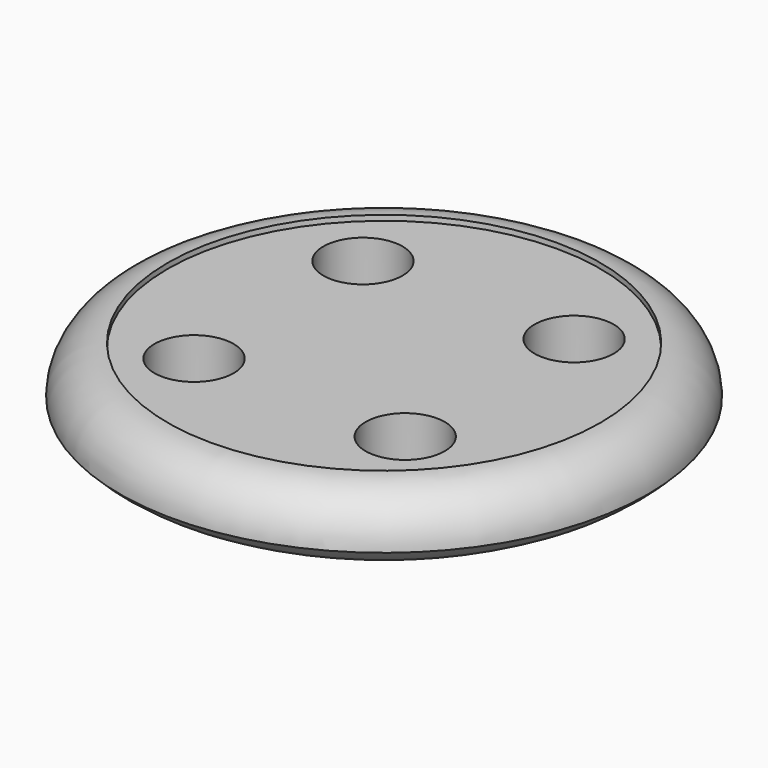
from build123d import *

# Parameters (mm, degrees)
F0_R     = 12.7
F0_R_2   = 1.905
F1_DEPTH = 1.905
F2_R     = 2.286
F4_DEPTH = 0.254
F5_DEPTH = 0.254


# Not quite as in the source:
# - a fillet or chamfer that OpenCascade refuses, or shapes differently, is made with other operations: its cross-section is extruded or revolved along the edge and cut away or added


with BuildPart() as f1:
    # F0 (on Top) → F1 (new body, symmetric)
    with BuildSketch(Plane.XY):
        Circle(F0_R)
        with Locations((-5.08, -5.08)):
            Circle(F0_R_2, mode=Mode.SUBTRACT)
        with Locations((5.08, -5.08)):
            Circle(F0_R_2, mode=Mode.SUBTRACT)
        with Locations((-5.08, 5.08)):
            Circle(F0_R_2, mode=Mode.SUBTRACT)
        with Locations((5.08, 5.08)):
            Circle(F0_R_2, mode=Mode.SUBTRACT)
    extrude(amount=F1_DEPTH, both=True)

    # F2
    f2_edges = [f1.edges().sort_by_distance(p)[0] for p in [
        (-12.7, 0, 1.905),
    ]]
    fillet(f2_edges, radius=F2_R)

    # F3: fillet of radius 4.826 on 1 edges, made by hand

    # F3_s1 → F3_t2 (revolve, cut)
    with BuildSketch(Plane.XZ):
        with BuildLine():
            ThreePointArc((12.7, -0.381), (11.0981307056, -1.5076413266), (9.180472759, -1.905))
            Line((9.180472759, -1.905), (12.7, -1.905))
            Line((12.7, -1.905), (12.7, -0.381))
        make_face()
    revolve(axis=Axis((0, 0, -1.905), (0, 0, 1)), mode=Mode.SUBTRACT)

    # F4 (cut): a face of the model
    f4_faces = [f1.faces().sort_by_distance(p)[0] for p in [
        (0, 0, 1.905),
    ]]
    extrude(f4_faces, amount=-F4_DEPTH, mode=Mode.SUBTRACT)

    # F5 (cut): a face of the model
    f5_faces = [f1.faces().sort_by_distance(p)[0] for p in [
        (0, 0, -1.905),
    ]]
    extrude(f5_faces, amount=-F5_DEPTH, mode=Mode.SUBTRACT)


solid = f1.part
